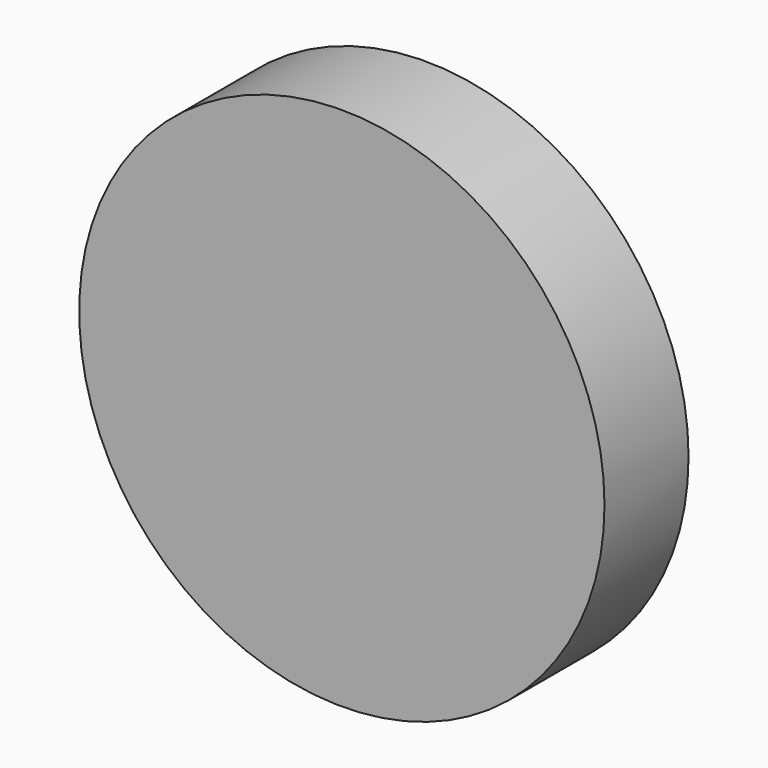
from build123d import *

# Parameters (mm, degrees)
F5_R     = 375
F5_R_2   = 370
F6_DEPTH = 150
F0_R     = 375


# Not quite as in the source:
# - a feature of the source that left no trace in its solid (it failed there, or was rolled back) is left out
# - the program builds the solid bodies; features that only make, move or delete a surface that nothing else refers to are left out


with BuildPart() as f6:
    # F5 (on face) → F6 (new body)
    with BuildSketch(Plane.XZ):
        Circle(F5_R)
        Circle(F5_R_2, mode=Mode.SUBTRACT)
    extrude(amount=F6_DEPTH)


with BuildPart() as f6b:
    # F0 (on Front) → F6, piece 2 (new body)
    with BuildSketch(Plane.XZ):
        Circle(F0_R)
    extrude(amount=F6_DEPTH)


solid = Compound([f6.part, f6b.part])
